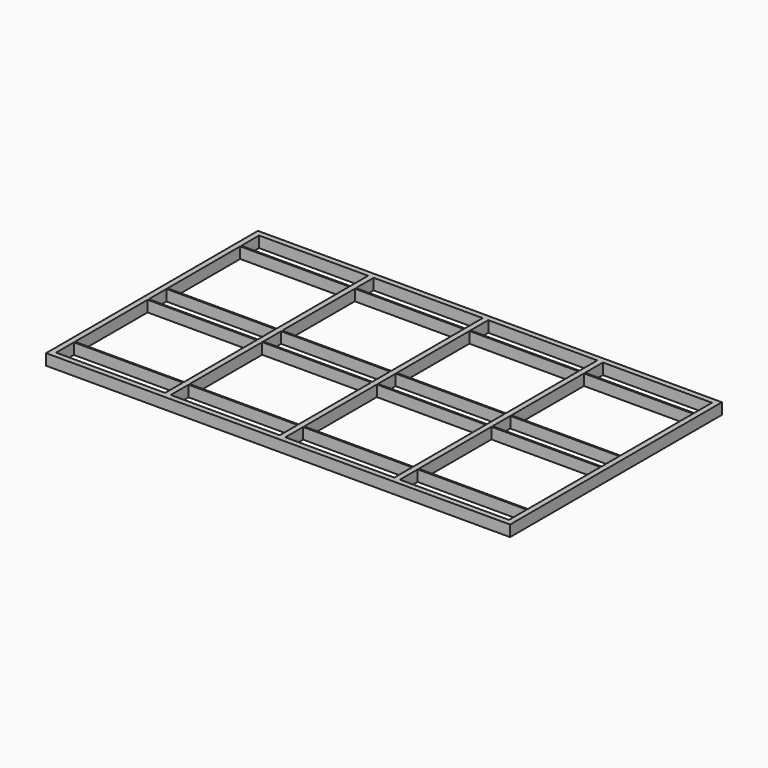
from build123d import *

# Parameters (mm, degrees)
F0_W     = 490
F0_H     = 6
F1_DEPTH = 50


# Not quite as in the source:
# - a feature names something its author has since deleted; it is built from what else it names
# - the program builds the solid bodies; features that only make, move or delete a surface that nothing else refers to are left out


with BuildPart() as f1:
    # F0 (on Top) → F1 (new body)
    with BuildSketch(Plane.XY):
        Polygon((0, 1190), (0, 0), (515, 0), (540, 0), (540, 25), (540, 125), (540, 131), (540, 539), (540, 545), (540, 645), (540, 651), (540, 1059), (540, 1065), (540, 1165), (540, 1190), (515, 1190), align=None)
        Polygon((25, 1065), (25, 1165), (515, 1165), (515, 1065), (515, 1059), (515, 651), (515, 645), (515, 545), (515, 539), (515, 131), (515, 125), (515, 25), (25, 25), (25, 125), (25, 131), (25, 539), (25, 545), (25, 645), (25, 651), (25, 1059), align=None, mode=Mode.SUBTRACT)
        Polygon((540, 25), (540, 0), (1030, 0), (1055, 0), (1055, 25), (1055, 125), (1055, 131), (1055, 539), (1055, 545), (1055, 645), (1055, 651), (1055, 1059), (1055, 1065), (1055, 1165), (1055, 1190), (1030, 1190), (540, 1190), (540, 1165), (1030, 1165), (1030, 1065), (1030, 1059), (1030, 651), (1030, 645), (1030, 545), (1030, 539), (1030, 131), (1030, 125), (1030, 25), align=None)
        Polygon((1055, 25), (1055, 0), (1545, 0), (1570, 0), (1570, 25), (1570, 125), (1570, 131), (1570, 539), (1570, 545), (1570, 645), (1570, 651), (1570, 1059), (1570, 1065), (1570, 1165), (1570, 1190), (1545, 1190), (1055, 1190), (1055, 1165), (1545, 1165), (1545, 1065), (1545, 1059), (1545, 651), (1545, 645), (1545, 545), (1545, 539), (1545, 131), (1545, 125), (1545, 25), align=None)
        Polygon((1570, 25), (1570, 0), (2085, 0), (2085, 1190), (1570, 1190), (1570, 1165), (2060, 1165), (2060, 1065), (2060, 1059), (2060, 651), (2060, 645), (2060, 545), (2060, 539), (2060, 131), (2060, 125), (2060, 25), align=None)
        with Locations((270, 542)):
            Rectangle(F0_W, F0_H)
        with Locations((270, 128)):
            Rectangle(F0_W, F0_H)
        with Locations((270, 648)):
            Rectangle(F0_W, F0_H)
        with Locations((270, 1062)):
            Rectangle(F0_W, F0_H)
        with Locations((785, 648)):
            Rectangle(F0_W, F0_H)
        with Locations((1300, 648)):
            Rectangle(F0_W, F0_H)
        with Locations((1300, 542)):
            Rectangle(F0_W, F0_H)
        with Locations((785, 542)):
            Rectangle(F0_W, F0_H)
        with Locations((1815, 542)):
            Rectangle(F0_W, F0_H)
        with Locations((1815, 648)):
            Rectangle(F0_W, F0_H)
        with Locations((1815, 1062)):
            Rectangle(F0_W, F0_H)
        with Locations((1300, 1062)):
            Rectangle(F0_W, F0_H)
        with Locations((785, 1062)):
            Rectangle(F0_W, F0_H)
        with Locations((1815, 128)):
            Rectangle(F0_W, F0_H)
        with Locations((785, 128)):
            Rectangle(F0_W, F0_H)
        with Locations((1300, 128)):
            Rectangle(F0_W, F0_H)
    extrude(amount=F1_DEPTH)


solid = f1.part
